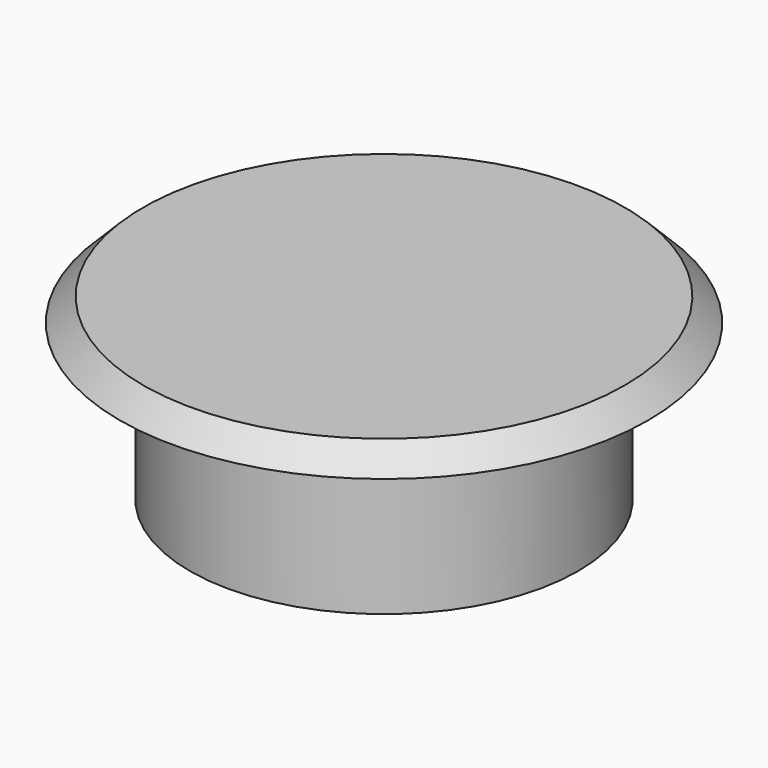
from build123d import *

# Parameters (mm, degrees)
F0_W = 1.5
F0_H = 10


# Not quite as in the source:
# - a fillet or chamfer that OpenCascade refuses, or shapes differently, is made with other operations: its cross-section is extruded or revolved along the edge and cut away or added


with BuildPart() as f1:
    # F0 (on Front) → F1 (revolve)
    with BuildSketch(Plane.XZ):
        Polygon((0, 11.5), (0, 10), (11, 10), (12.5, 10), (17.5, 10), (17.5, 11.5), align=None)
        with Locations((11.75, 5)):
            Rectangle(F0_W, F0_H)
    revolve(axis=Axis((0, 0, 10.75), (0, 0, -1)))

    # F2: chamfer of 2 on 1 edges, made by hand

    # F2_s1 → F2_t2 (revolve, cut)
    with BuildSketch(Plane.XZ):
        Polygon((17.5, 9.5), (15.5, 11.5), (17.5, 11.5), align=None)
    revolve(axis=Axis((0, 0, 11.5), (0, 0, -1)), mode=Mode.SUBTRACT)


solid = f1.part
